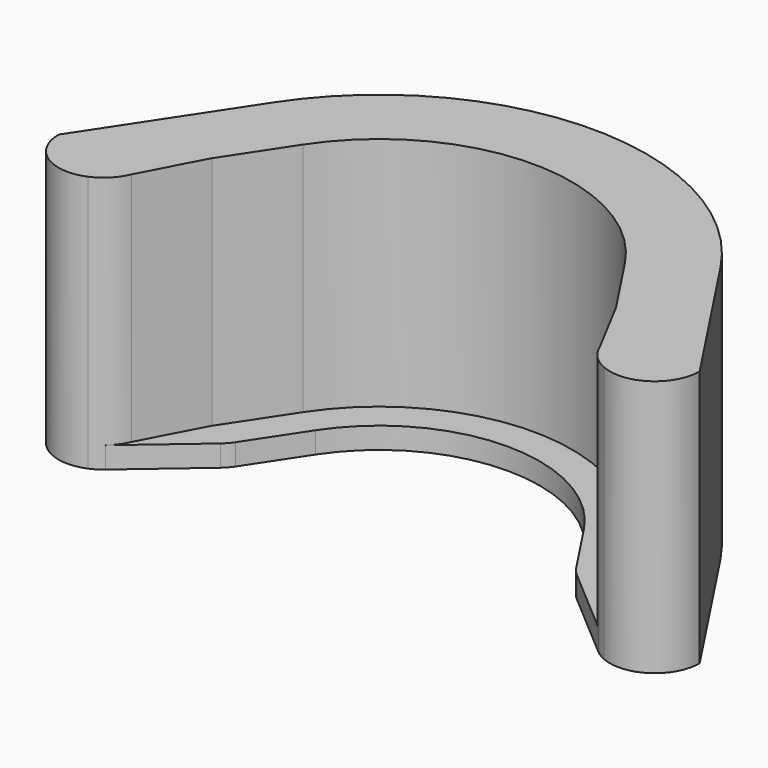
from build123d import *

# Parameters (mm, degrees)
F1_DEPTH    = 12
F2_W        = 1.5
F2_H        = 6
F3_DEPTH    = 12.5
F4_R        = 0.6
F5_T1_DEPTH = 12
F7_DEPTH    = 1


# Not quite as in the source:
# - a fillet or chamfer that OpenCascade refuses, or shapes differently, is made with other operations: its cross-section is extruded or revolved along the edge and cut away or added


with BuildPart() as f1:
    # F0 (on Top) → F1 (new body)
    with BuildSketch(Plane.XY):
        with BuildLine():
            ThreePointArc((-7.5164818898, 24.95), (0, 29), (7.5164818898, 24.95))
            Line((7.5164818898, 24.95), (10.7763181216, 20))
            Line((10.7763181216, 20), (14.9671085022, 20))
            Line((14.9671085022, 20), (10.4395581803, 26.875))
            ThreePointArc((10.4395581803, 26.875), (0, 32.5), (-10.4395581803, 26.875))
            Line((-10.4395581803, 26.875), (-13.6993944121, 21.925))
            ThreePointArc((-13.6993944121, 21.925), (-11.7192459572, 21.75), (-10.7763181216, 20))
            Line((-10.7763181216, 20), (-7.5164818898, 24.95))
        make_face()
        with BuildLine():
            Line((14.9671085022, 20), (10.7763181216, 20))
            Line((10.7763181216, 20), (12.0440322117, 18.075))
            ThreePointArc((12.0440322117, 18.075), (14.0241806666, 18.25), (14.9671085022, 20))
        make_face()
        with BuildLine():
            Line((12.0440322117, 18.075), (10.7763181216, 20))
            ThreePointArc((10.7763181216, 20), (11.1217133119, 18.8475326453), (12.0440322117, 18.075))
        make_face()
        with BuildLine():
            ThreePointArc((-12.0440322117, 18.075), (-11.1217133119, 18.8475326453), (-10.7763181216, 20))
            Line((-10.7763181216, 20), (-12.0440322117, 18.075))
        make_face()
        with BuildLine():
            Line((-12.0440322117, 18.075), (-10.7763181216, 20))
            Line((-10.7763181216, 20), (-14.9671085022, 20))
            ThreePointArc((-14.9671085022, 20), (-14.0241806666, 18.25), (-12.0440322117, 18.075))
        make_face()
        with BuildLine():
            Line((-14.9671085022, 20), (-10.7763181216, 20))
            ThreePointArc((-10.7763181216, 20), (-11.7192459572, 21.75), (-13.6993944121, 21.925))
            Line((-13.6993944121, 21.925), (-14.9671085022, 20))
        make_face()
    extrude(amount=F1_DEPTH)

    # F2 (on Right) → F3 (cut, symmetric)
    with BuildSketch(Plane.YZ):
        with Locations((31.75, 6)):
            Rectangle(F2_W, F2_H)
    extrude(amount=F3_DEPTH, both=True, mode=Mode.SUBTRACT)

    # F4
    f4_edges = [f1.edges().sort_by_distance(p)[0] for p in [
        (0, 31, 9),
        (0, 31, 3),
    ]]
    fillet(f4_edges, radius=F4_R)

    # F5: chamfer of 5 on 2 edges, made by hand

    # F5_s2 → F5_t1 (join)
    with BuildSketch(Plane.XY):
        with BuildLine():
            Line((11.0273555293, 19.0260146009), (9.3449019992, 22.2084505142))
            Line((9.3449019992, 22.2084505142), (9.4284184646, 22.2634505142))
            ThreePointArc((9.4284184646, 22.2634505142), (10.1361174506, 21.1539508584), (10.859834587, 20.055))
            Line((10.859834587, 20.055), (10.8763181216, 20))
            ThreePointArc((10.8763181216, 20), (10.9346351532, 19.5211157003), (11.1198360632, 19.0640586655))
            Line((11.1198360632, 19.0640586655), (11.0273555293, 19.0260146009))
        make_face()
        with BuildLine():
            Line((-9.3449019992, 22.2084505142), (-11.0273555293, 19.0260146009))
            Line((-11.0273555293, 19.0260146009), (-11.1198360632, 19.0640586655))
            ThreePointArc((-11.1198360632, 19.0640586655), (-10.9346351532, 19.5211157003), (-10.8763181216, 20))
            Line((-10.8763181216, 20), (-10.859834587, 20.055))
            ThreePointArc((-10.859834587, 20.055), (-10.1361174506, 21.1539508584), (-9.4284184646, 22.2634505142))
            Line((-9.4284184646, 22.2634505142), (-9.3449019992, 22.2084505142))
        make_face()
    extrude(amount=F5_T1_DEPTH)

    # F6 (on face) → F7 (join)
    with BuildSketch(Plane(origin=(0, 0, 0), x_dir=(1, 0, 0), z_dir=(0, 0, -1))):
        with BuildLine():
            ThreePointArc((-7.5164818898, -24.95), (0, -29), (7.5164818898, -24.95))
            Line((7.5164818898, -24.95), (9.4383768754, -22.0316386155))
            Line((9.4383768756, -22.0316386152), (10.9338806529, -19.2028264998))
            ThreePointArc((10.9338806529, -19.2028264998), (11.1736784475, -18.772254667), (11.507412541, -18.4096024365))
            Line((11.507412541, -18.4096024365), (8.3196064123, -21.1442182701))
            ThreePointArc((8.3196064123, -21.1442182701), (8.1209139726, -21.3403362232), (7.9514665684, -21.5622112204))
            Line((7.9514665684, -21.5622112204), (6.2637349082, -24.125))
            ThreePointArc((6.2637349082, -24.125), (0, -27.5), (-6.2637349082, -24.125))
            Line((-6.2637349082, -24.125), (-7.9514665684, -21.5622112204))
            ThreePointArc((-7.9514665684, -21.5622112204), (-8.1209139726, -21.3403362232), (-8.3196064123, -21.1442182701))
            Line((-8.3196064123, -21.1442182701), (-11.507412541, -18.4096024365))
            ThreePointArc((-11.507412541, -18.4096024365), (-11.1736784475, -18.772254667), (-10.9338806529, -19.2028264998))
            Line((-10.9338806529, -19.2028264998), (-9.4383768756, -22.0316386152))
            Line((-9.4383768756, -22.0316386152), (-7.5164818898, -24.95))
        make_face()
    extrude(amount=-F7_DEPTH)


solid = f1.part
